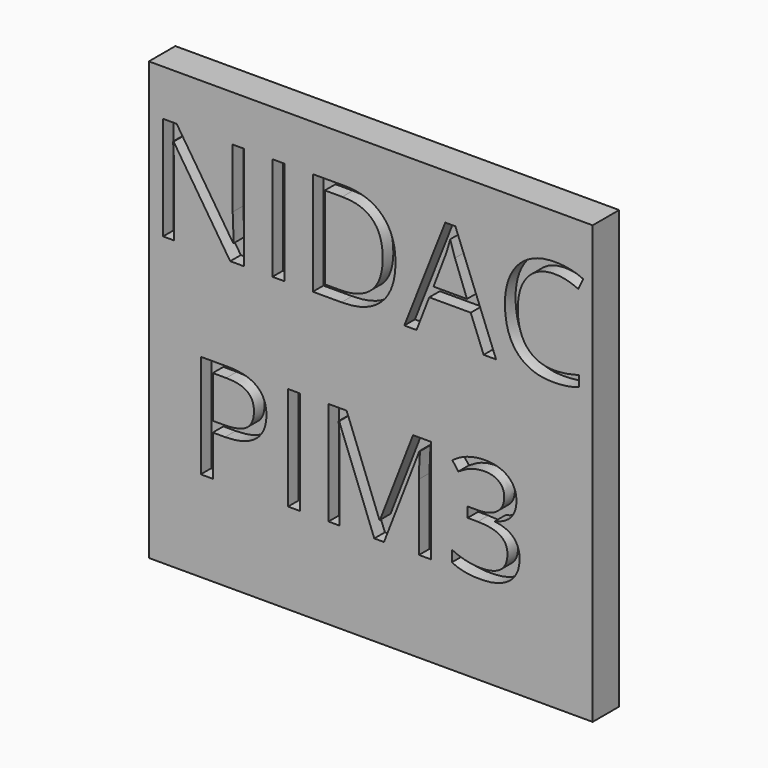
from build123d import *

# Parameters (mm, degrees)
F0_W         = 67
F0_H         = 66
F1_DEPTH     = 5
F2_TEXT_SIZE = 21.8920712718
F3_DEPTH     = 2


# Not quite as in the source:
# - Text() gives the source's letters only with a copy of the font that has no kerning and outlines rounded to 1/6400 em; it was checked with that copy


with BuildPart() as f1:
    # F0 (on Front) → F1 (new body)
    with BuildSketch(Plane.XZ):
        Rectangle(F0_W, F0_H)
    extrude(amount=F1_DEPTH)

    # F2 (on face) → F3 (cut)
    with BuildSketch(Plane.XZ.offset(5)):
        with Locations((-33.5, 10.4372434853)):
            Text('NIDAC', F2_TEXT_SIZE, font='Open Sans', text_align=(TextAlign.LEFT, TextAlign.BOTTOM))
        with Locations((-27.8114821055, -19.3359734443)):
            Text('PIM3', F2_TEXT_SIZE, font='Open Sans', text_align=(TextAlign.LEFT, TextAlign.BOTTOM))
    extrude(amount=-F3_DEPTH, mode=Mode.SUBTRACT)


solid = f1.part
